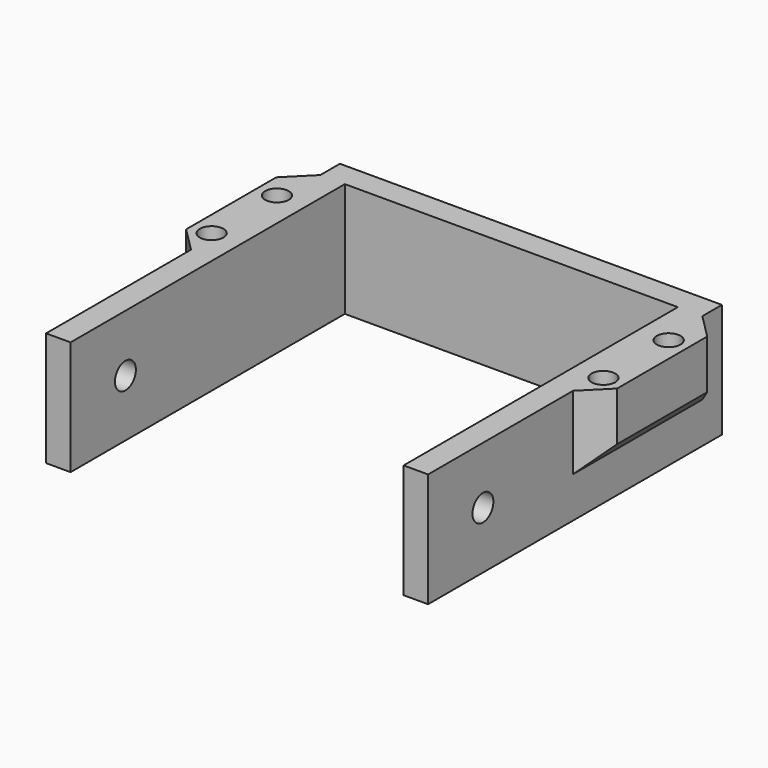
from build123d import *

# Parameters (mm, degrees)
F1_DEPTH = 14
F2_W     = 6
F2_H     = 19.8
F3_DEPTH = 9
F4_R     = 1.45
F5_DEPTH = 6.5
F6_SIZE  = 2.99999
F7_R     = 1.6
F8_DEPTH = 3
F10_SIZE = 1.45


# Not quite as in the source:
# - a fillet or chamfer is up to 0.001 mm smaller than in the source, because OpenCascade refuses the exact size


with BuildPart() as f1:
    # F0 (on Top) → F1 (new body)
    with BuildSketch(Plane.XY):
        Polygon((0, 24.2671520197), (0, 21.2671520197), (20.4, 21.2671520197), (20.4, -20.7328479803), (23.4, -20.7328479803), (23.4, 24.2671520197), align=None)
    extrude(amount=F1_DEPTH)

    # F2 (on face) → F3 (join)
    with BuildSketch(Plane.XY.offset(14)):
        with Locations((23.4, 11.3671520197)):
            Rectangle(F2_W, F2_H)
    extrude(amount=-F3_DEPTH)

    # F4 (on face) → F5 (cut)
    with BuildSketch(Plane.XY.offset(14)):
        with Locations((24, 5.3671520197)):
            Circle(F4_R)
        with Locations((24, 15.3671520197)):
            Circle(F4_R)
    extrude(amount=-F5_DEPTH, mode=Mode.SUBTRACT)

    # F6 (size 3 in the source; OpenCascade refuses exactly that, so slightly less here)
    f6_edges = [f1.edges().sort_by_distance(p)[0] for p in [
        (26.4, 1.467152, 9.5),
        (26.4, 21.267152, 9.5),
        (26.4, 11.367152, 5),
    ]]
    chamfer(f6_edges, length=F6_SIZE)

    # F7 (on face) → F8 (cut, through all)
    with BuildSketch(Plane.YZ.offset(23.4)):
        with Locations((-12.3328479803, 7)):
            Circle(F7_R)
    extrude(amount=-F8_DEPTH, mode=Mode.SUBTRACT)

    # F9: F1 across plane


with BuildPart() as f1_1:
    add(f1.part)
    add(f1.part.mirror(Plane.YZ))

    # F10
    f10_edges = [f1_1.edges().sort_by_distance(p)[0] for p in [
        (22.55, 15.367152, 7.5),
        (22.55, 5.367152, 7.5),
        (-22.55, 5.367152, 7.5),
        (-22.55, 15.367152, 7.5),
    ]]
    chamfer(f10_edges, length=F10_SIZE)


solid = f1_1.part
